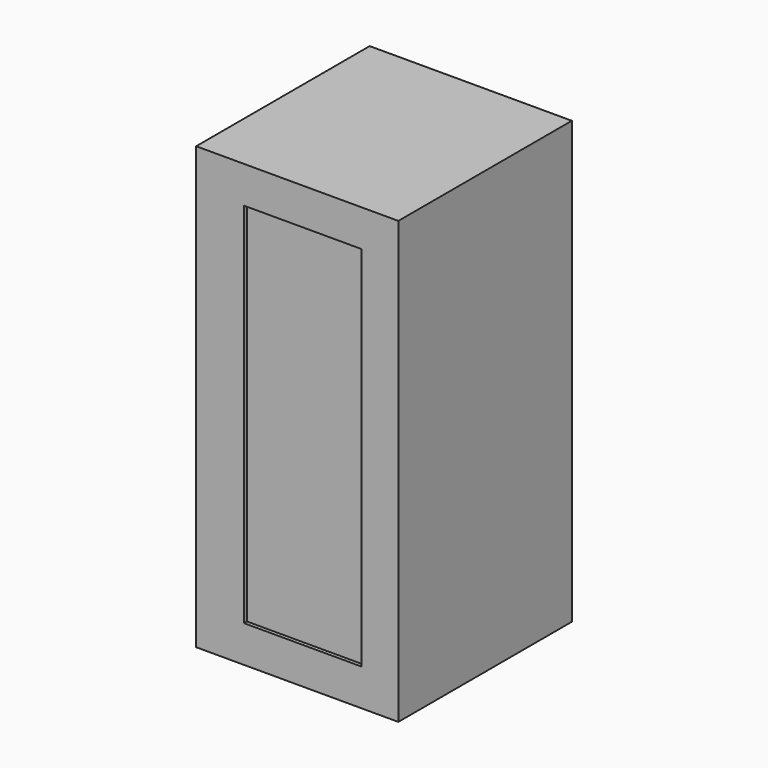
from build123d import *

# Parameters (mm, degrees)
F0_W     = 330.2
F0_H     = 762
F0_W_2   = 203.2
F0_H_2   = 635
F1_DEPTH = 374.65
F2_DEPTH = 6.35
F3_W     = 374.65
F3_H     = 762
F3_W_2   = 247.65
F3_H_2   = 635
F4_DEPTH = 19.05
F5_DEPTH = 12.7


# Not quite as in the source:
# - a feature names something its author has since deleted; it is built from what else it names


with BuildPart() as f1:
    # F0 (on Front) → F1 (new body)
    with BuildSketch(Plane.XZ):
        with Locations((48.0267770052, 381)):
            Rectangle(F0_W, F0_H)
        with Locations((48.0267770052, 381)):
            Rectangle(F0_W_2, F0_H_2, mode=Mode.SUBTRACT)
        with Locations((48.0267770052, 381)):
            Rectangle(F0_W_2, F0_H_2)
    extrude(amount=-F1_DEPTH)

    # F0 (on Front) → F2 (cut)
    with BuildSketch(Plane.XZ):
        with Locations((48.0267770052, 381)):
            Rectangle(F0_W_2, F0_H_2)
    extrude(amount=-F2_DEPTH, mode=Mode.SUBTRACT)

    # F3 (on face) → F4 (join)
    with BuildSketch(Plane(origin=(-117.0732229948, 0, 0), x_dir=(0, -1, 0), z_dir=(-1, 0, 0))):
        with Locations((-187.325, 381)):
            Rectangle(F3_W, F3_H)
        with Locations((-187.325, 381)):
            Rectangle(F3_W_2, F3_H_2, mode=Mode.SUBTRACT)
    extrude(amount=F4_DEPTH)

    # F5 (add): a face of the model
    f5_faces = [f1.faces().sort_by_distance(p)[0] for p in [
        (-117.0732229948, 187.325, 381),
    ]]
    extrude(f5_faces, amount=F5_DEPTH)


solid = f1.part
